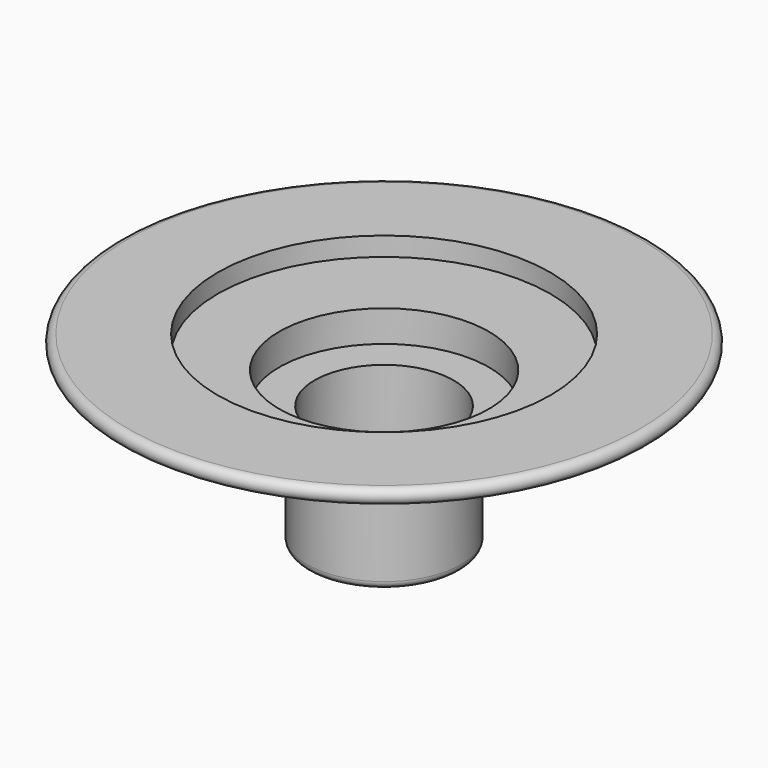
from build123d import *

# Parameters (mm, degrees)
F2_T     = 2.54
F3_R     = 2.54
F4_SIZE  = 5.08
F5_W     = 8.4462584928
F5_H     = 4.5507363975
F6_DEPTH = 2.54
F7_T     = -0.254
F7_2_T   = -0.254
F8_DEPTH = 12.7


# Not quite as in the source:
# - a shell that OpenCascade refuses in one call is made with other operations: the cavity is built on its own and cut out


with BuildPart() as f1:
    # F0 (on Right) → F1 (revolve)
    with BuildSketch(Plane.YZ):
        Polygon((-55.6017309427, 0), (-98.8910123706, 0), (-65.6718313694, -13.2572650909), (-37.5815480947, -13.2572650909), (-37.5815480947, -23.7286388874), (-25.7504582405, -23.7286388874), (-25.7504582405, -62.0390437543), (0, -62.0390437543), (0, -6.2905848026), (-55.6017309427, -6.2905848026), align=None)
    revolve(axis=Axis((0, 0, 15.0363594294), (0, 0, 1)))

    # F2: shell of thickness 2.54, made by hand


with BuildPart() as f2_core1:
    # F2_t2: copy of F1
    add(f1.part)

    # the walls: a layer under each face that stays
    f2_faces = [f2_core1.faces().sort_by_distance(p)[0] for p in [
        (0, 55.6017309427, -3.1452924013),
        (-65.9273415804, -65.9273415804, 0),
        (0, 82.28142187, -6.6286325455),
        (-43.7812209129, 43.7812209129, -13.2572650909),
        (0, 37.5815480947, -18.4929519892),
        (-25.0543653965, 25.0543653965, -23.7286388874),
        (0, 25.7504582405, -42.8838413209),
        (0, 0, -62.0390437543),
    ]]
    thicken(f2_faces, amount=-F2_T, mode=Mode.SUBTRACT)

    # F2_s3 → F2_t4 (revolve, cut)
    with BuildSketch(Plane.YZ):
        Polygon((-37.6069480947, -13.2826650909), (-37.5815480947, -10.7172650909), (-35.0415480947, -10.7172650909), (-35.0415480947, -13.2572650909), align=None)
    revolve(axis=Axis((0, 0, -13.2572650909), (0, 0, 1)), mode=Mode.SUBTRACT)

    # F2_s5 → F2_t6 (revolve, cut)
    with BuildSketch(Plane.YZ):
        Polygon((-25.7758582405, -23.7540388874), (-25.7504582405, -21.1886388874), (-23.2104582405, -21.1886388874), (-23.2104582405, -23.7286388874), align=None)
    revolve(axis=Axis((0, 0, -23.7286388874), (0, 0, 1)), mode=Mode.SUBTRACT)


with BuildPart() as f1_1:
    add(f1.part)

    # what is left inside the walls is the cavity
    f2_cavity = [f2_core1.part.solids().sort_by_distance(p)[0] for p in [
        (-66.635149, 42.836882, -2.5654),
    ]]
    add(f2_cavity, mode=Mode.SUBTRACT)

    # F3
    f3_edges = [f1_1.edges().sort_by_distance(p)[0] for p in [
        (0, 25.750458, -62.039044),
        (0, 25.750458, -23.728639),
        (0, 37.581548, -13.257265),
        (0, 37.581548, -23.728639),
        (0, 65.671831, -13.257265),
        (0, 98.891012, 0),
    ]]
    fillet(f3_edges, radius=F3_R)

    # F4
    f4_edges = [f1_1.edges().sort_by_distance(p)[0] for p in [
        (0, 23.210458, -59.499044),
    ]]
    chamfer(f4_edges, length=F4_SIZE)


with BuildPart() as f6:
    # F5 (on face) → F6 (new body)
    with BuildSketch(Plane(origin=(0, 0, -62.0390437543), x_dir=(1, 0, 0), z_dir=(0, 0, -1))):
        with Locations((13.5994190318, 2.2753681988)):
            Rectangle(F5_W, F5_H)
    extrude(amount=F6_DEPTH)

    # F7#2
    f7_2_openings = [f6.faces().sort_by_distance(p)[0] for p in [
        (13.599419, 0, -63.309044),
    ]]
    offset(amount=F7_2_T, openings=f7_2_openings)


with BuildPart() as f6b:
    # F5 (on face) → F6, piece 2 (new body)
    with BuildSketch(Plane(origin=(0, 0, -62.0390437543), x_dir=(1, 0, 0), z_dir=(0, 0, -1))):
        with Locations((-4.2231292464, 2.2753681988)):
            Rectangle(F5_W, F5_H)
    extrude(amount=F6_DEPTH)

    # F7
    f7_openings = [f6b.faces().sort_by_distance(p)[0] for p in [
        (-4.223129, 0, -63.309044),
    ]]
    offset(amount=F7_T, openings=f7_openings)


with BuildPart() as f8:
    # F8 (new): a face of the model
    f8_faces = [f6.part.faces().sort_by_distance(p)[0] for p in [
        (13.5994190318, -4.2967363975, -63.3090437543),
    ]]
    extrude(f8_faces, amount=F8_DEPTH)


with BuildPart() as f8b:
    # F8#2 (new): a face of the model
    f8_2_faces = [f6b.part.faces().sort_by_distance(p)[0] for p in [
        (-4.2231292464, -4.2967363975, -63.3090437543),
    ]]
    extrude(f8_2_faces, amount=F8_DEPTH)


solid = Compound([f1_1.part, f6.part, f6b.part, f8.part, f8b.part])
